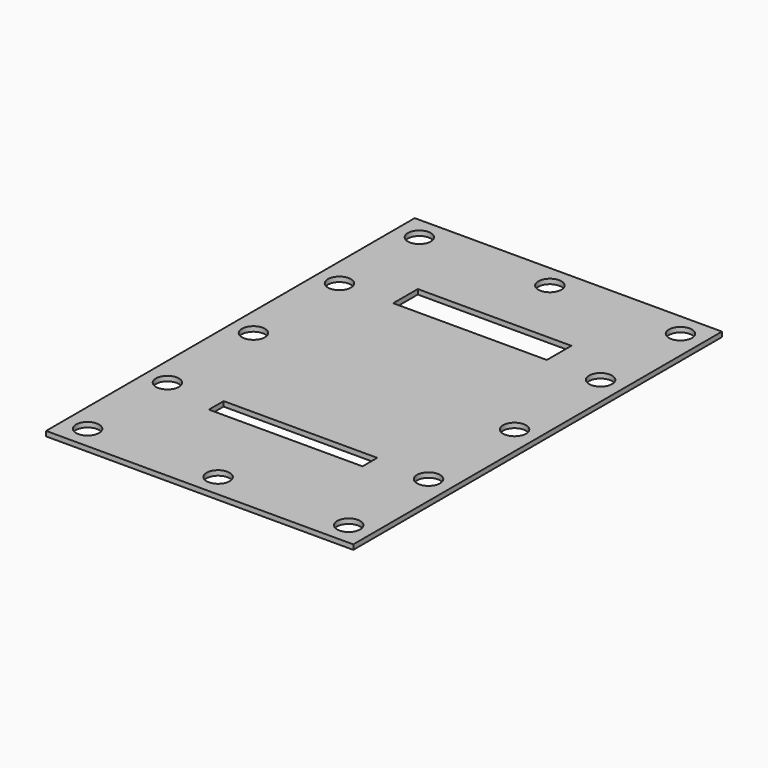
from build123d import *

# Parameters (mm, degrees)
F0_W     = 100
F0_H     = 150
F1_DEPTH = 1.5875
F2_R     = 3.75
F3_DEPTH = 25
F4_W     = 50
F4_H     = 6
F5_DEPTH = 25
F6_W     = 50
F6_H     = 10
F7_DEPTH = 25


# Not quite as in the source:
# - a feature names something its author has since deleted; it is built from what else it names


with BuildPart() as f1:
    # F0 (on Top) → F1 (new body)
    with BuildSketch(Plane.XY):
        Rectangle(F0_W, F0_H)
    extrude(amount=F1_DEPTH)

    # F2 (on face) → F3 (cut)
    with BuildSketch(Plane.XY.offset(1.5875)):
        with Locations((-42.5, 67.5)):
            Circle(F2_R)
        with Locations((-42.5, 0)):
            Circle(F2_R)
        with Locations((-42.5, -35)):
            Circle(F2_R)
        with Locations((-42.5, -67.5)):
            Circle(F2_R)
        with Locations((0, -67.5)):
            Circle(F2_R)
        with Locations((-42.5, 35)):
            Circle(F2_R)
        with Locations((42.5, -67.5)):
            Circle(F2_R)
        with Locations((42.5, -35)):
            Circle(F2_R)
        with Locations((42.5, 0)):
            Circle(F2_R)
        with Locations((42.5, 35)):
            Circle(F2_R)
        with Locations((42.5, 67.5)):
            Circle(F2_R)
        with Locations((0, 67.5)):
            Circle(F2_R)
    extrude(amount=-F3_DEPTH, mode=Mode.SUBTRACT)

    # F4 (on face) → F5 (cut)
    with BuildSketch(Plane.XY.offset(1.5875)):
        with Locations((0, -37)):
            Rectangle(F4_W, F4_H)
    extrude(amount=-F5_DEPTH, mode=Mode.SUBTRACT)

    # F6 (on face) → F7 (cut)
    with BuildSketch(Plane.XY.offset(1.5875)):
        with Locations((0, 40)):
            Rectangle(F6_W, F6_H)
    extrude(amount=-F7_DEPTH, mode=Mode.SUBTRACT)


solid = f1.part
